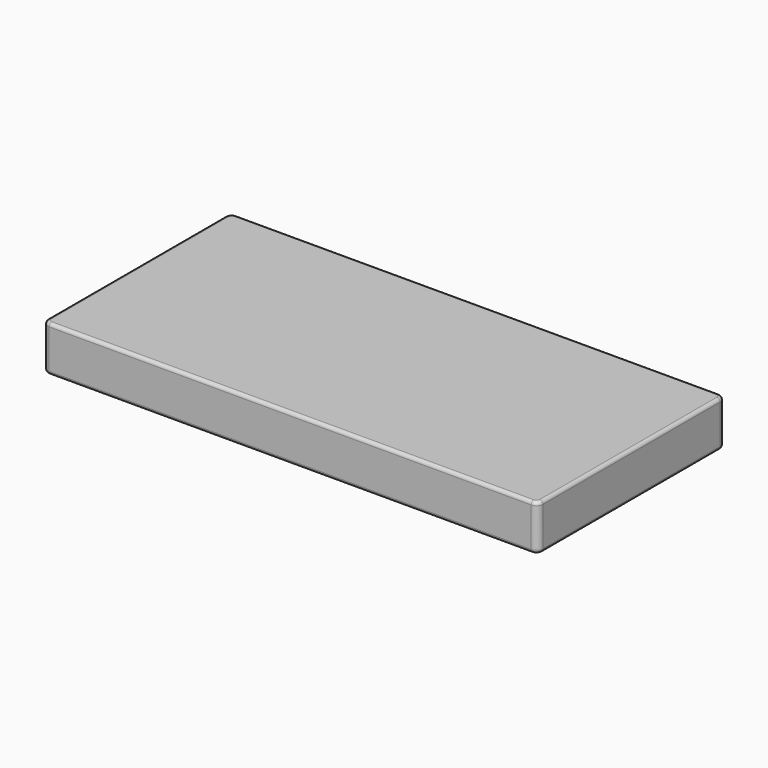
from build123d import *

# Parameters (mm, degrees)
F0_W         = 1930.4
F0_H         = 914.4
F1_DEPTH     = 177.8
F2_R         = 12.7
F3_R         = 12.7
F4_T1_DEPTH  = 177.8
F4_T4_ANGLE  = 90
F4_T6_ANGLE  = 90
F4_T8_ANGLE  = 90
F4_T10_ANGLE = 90
F4_T12_ANGLE = 90
F4_T14_ANGLE = 90
F4_T16_ANGLE = 90
F4_T18_ANGLE = 90


# Not quite as in the source:
# - a fillet or chamfer that OpenCascade refuses, or shapes differently, is made with other operations: its cross-section is extruded or revolved along the edge and cut away or added


with BuildPart() as f1:
    # F0 (on Top) → F1 (new body)
    with BuildSketch(Plane.XY):
        with Locations((-965.2, 457.2)):
            Rectangle(F0_W, F0_H)
    extrude(amount=F1_DEPTH)

    # F2
    f2_edges = [f1.edges().sort_by_distance(p)[0] for p in [
        (-965.2, 0, 177.8),
        (0, 457.2, 177.8),
        (-965.2, 914.4, 177.8),
        (-1930.4, 457.2, 177.8),
    ]]
    fillet(f2_edges, radius=F2_R)

    # F3
    f3_edges = [f1.edges().sort_by_distance(p)[0] for p in [
        (-965.2, 0, 0),
        (0, 457.2, 0),
        (-965.2, 914.4, 0),
        (-1930.4, 457.2, 0),
    ]]
    fillet(f3_edges, radius=F3_R)

    # F4: fillet of radius 25.4 on 4 edges, made by hand

    # F4_s2 → F4_t1 (cut)
    with BuildSketch(Plane.XY):
        with BuildLine():
            ThreePointArc((-1930.4, 889), (-1922.9605122421, 906.9605122421), (-1905, 914.4))
            Line((-1905, 914.4), (-1930.4, 914.4))
            Line((-1930.4, 914.4), (-1930.4, 889))
        make_face()
        with BuildLine():
            ThreePointArc((-1905, 0), (-1922.9605122421, 7.4394877579), (-1930.4, 25.4))
            Line((-1930.4, 25.4), (-1930.4, 0))
            Line((-1930.4, 0), (-1905, 0))
        make_face()
        with BuildLine():
            ThreePointArc((-25.4, 0), (-7.4394877579, 7.4394877579), (0, 25.4))
            Line((0, 25.4), (0, 0))
            Line((0, 0), (-25.4, 0))
        make_face()
        with BuildLine():
            ThreePointArc((0, 889), (-7.4394877579, 906.9605122421), (-25.4, 914.4))
            Line((-25.4, 914.4), (0, 914.4))
            Line((0, 914.4), (0, 889))
        make_face()
    extrude(amount=F4_T1_DEPTH, mode=Mode.SUBTRACT)

    # F4_s3 → F4_t4 (revolve, cut)
    with BuildSketch(Plane.YZ.offset(-25.4)):
        with BuildLine():
            ThreePointArc((901.7, 0), (910.6802561211, 3.7197438789), (914.4, 12.7))
            Line((914.4, 12.7), (914.4, 0))
            Line((914.4, 0), (901.7, 0))
        make_face()
    revolve(axis=Axis((-25.4, 889, 0), (0, 0, -1)), revolution_arc=F4_T4_ANGLE, mode=Mode.SUBTRACT)

    # F4_s5 → F4_t6 (revolve, cut)
    with BuildSketch(Plane.XZ.offset(-889)):
        with BuildLine():
            ThreePointArc((-12.7, 177.8), (-3.7197438789, 174.0802561211), (0, 165.1))
            Line((0, 165.1), (0, 177.8))
            Line((0, 177.8), (-12.7, 177.8))
        make_face()
    revolve(axis=Axis((-25.4, 889, 177.8), (0, 0, 1)), revolution_arc=F4_T6_ANGLE, mode=Mode.SUBTRACT)

    # F4_s7 → F4_t8 (revolve, cut)
    with BuildSketch(Plane.XZ.offset(-25.4)):
        with BuildLine():
            ThreePointArc((-12.7, 0), (-3.7197438789, 3.7197438789), (0, 12.7))
            Line((0, 12.7), (0, 0))
            Line((0, 0), (-12.7, 0))
        make_face()
    revolve(axis=Axis((-25.4, 25.4, 0), (0, 0, -1)), revolution_arc=F4_T8_ANGLE, mode=Mode.SUBTRACT)

    # F4_s9 → F4_t10 (revolve, cut)
    with BuildSketch(Plane.YZ.offset(-25.4)):
        with BuildLine():
            ThreePointArc((12.7, 177.8), (3.7197438789, 174.0802561211), (0, 165.1))
            Line((0, 165.1), (0, 177.8))
            Line((0, 177.8), (12.7, 177.8))
        make_face()
    revolve(axis=Axis((-25.4, 25.4, 177.8), (0, 0, 1)), revolution_arc=F4_T10_ANGLE, mode=Mode.SUBTRACT)

    # F4_s11 → F4_t12 (revolve, cut)
    with BuildSketch(Plane.YZ.offset(-1905)):
        with BuildLine():
            ThreePointArc((12.7, 0), (3.7197438789, 3.7197438789), (0, 12.7))
            Line((0, 12.7), (0, 0))
            Line((0, 0), (12.7, 0))
        make_face()
    revolve(axis=Axis((-1905, 25.4, 0), (0, 0, -1)), revolution_arc=F4_T12_ANGLE, mode=Mode.SUBTRACT)

    # F4_s13 → F4_t14 (revolve, cut)
    with BuildSketch(Plane.XZ.offset(-25.4)):
        with BuildLine():
            ThreePointArc((-1917.7, 177.8), (-1926.6802561211, 174.0802561211), (-1930.4, 165.1))
            Line((-1930.4, 165.1), (-1930.4, 177.8))
            Line((-1930.4, 177.8), (-1917.7, 177.8))
        make_face()
    revolve(axis=Axis((-1905, 25.4, 177.8), (0, 0, 1)), revolution_arc=F4_T14_ANGLE, mode=Mode.SUBTRACT)

    # F4_s15 → F4_t16 (revolve, cut)
    with BuildSketch(Plane.XZ.offset(-889)):
        with BuildLine():
            ThreePointArc((-1917.7, 0), (-1926.6802561211, 3.7197438789), (-1930.4, 12.7))
            Line((-1930.4, 12.7), (-1930.4, 0))
            Line((-1930.4, 0), (-1917.7, 0))
        make_face()
    revolve(axis=Axis((-1905, 889, 0), (0, 0, -1)), revolution_arc=F4_T16_ANGLE, mode=Mode.SUBTRACT)

    # F4_s17 → F4_t18 (revolve, cut)
    with BuildSketch(Plane.YZ.offset(-1905)):
        with BuildLine():
            ThreePointArc((901.7, 177.8), (910.6802561211, 174.0802561211), (914.4, 165.1))
            Line((914.4, 165.1), (914.4, 177.8))
            Line((914.4, 177.8), (901.7, 177.8))
        make_face()
    revolve(axis=Axis((-1905, 889, 177.8), (0, 0, 1)), revolution_arc=F4_T18_ANGLE, mode=Mode.SUBTRACT)


solid = f1.part
